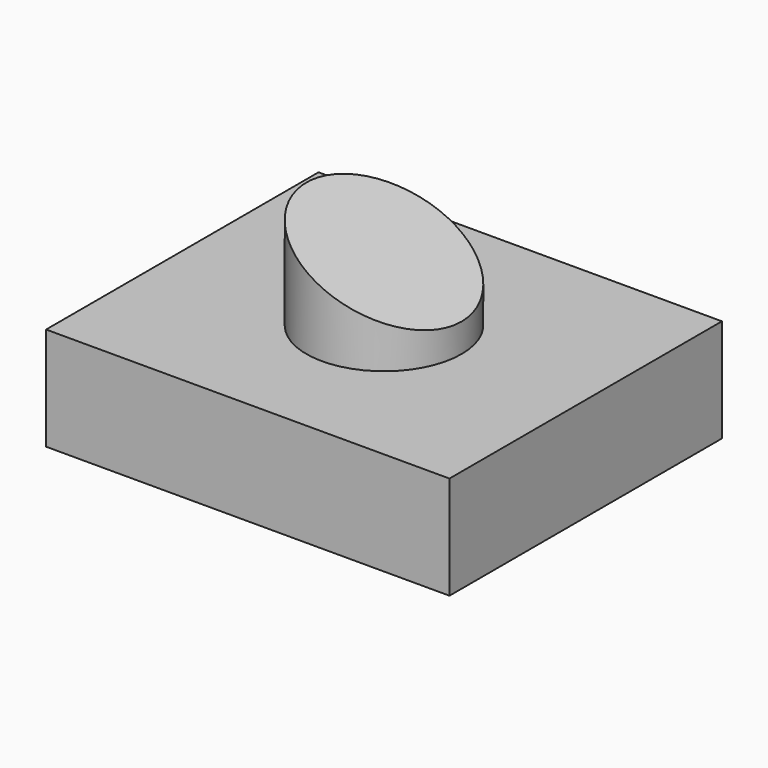
from build123d import *

# Parameters (mm, degrees)
F0_W     = 99.3201732635
F0_H     = 83.8441029191
F1_DEPTH = 25.4
F2_R     = 19.0950766662
F3_DEPTH = 25.4
F5_DEPTH = 44.35832


with BuildPart() as f1:
    # F0 (on Top) → F1 (new body)
    with BuildSketch(Plane.XY):
        Rectangle(F0_W, F0_H)
    extrude(amount=F1_DEPTH)

    # F2 (on face) → F3 (join)
    with BuildSketch(Plane.XY.offset(25.4)):
        Circle(F2_R)
    extrude(amount=F3_DEPTH)

    # F4 (on Front) → F5 (cut, symmetric)
    with BuildSketch(Plane.XZ):
        Polygon((21.8941513449, 53.4225776792), (-26.0670147836, 53.4225776792), (21.8941513449, 31.1297103763), align=None)
    extrude(amount=F5_DEPTH, both=True, mode=Mode.SUBTRACT)


solid = f1.part
